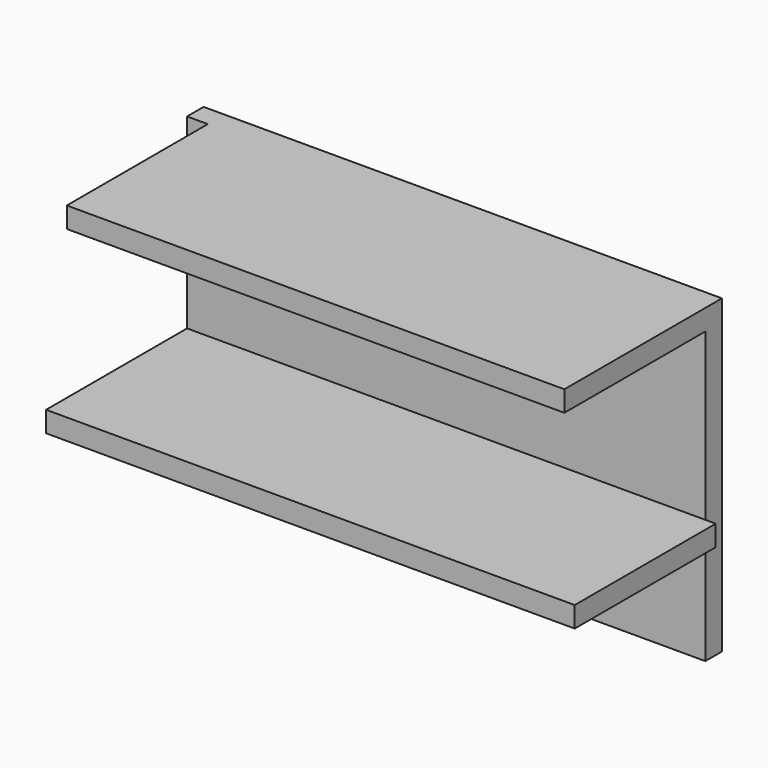
from build123d import *

# Parameters (mm, degrees)
F0_W     = 480
F0_H     = 190
F1_DEPTH = 20
F2_W     = 500
F2_H     = 300
F3_DEPTH = 20
F4_W     = 10
F4_H     = 20
F4_W_2   = 500
F5_DEPTH = 170


# Not quite as in the source:
# - the program builds the solid bodies; features that only make, move or delete a surface that nothing else refers to are left out


with BuildPart() as f1:
    # F0 (on Top) → F1 (new body)
    with BuildSketch(Plane.XY):
        with Locations((10, -95)):
            Rectangle(F0_W, F0_H)
    extrude(amount=-F1_DEPTH)

    # F2 (on Front) → F3 (join)
    with BuildSketch(Plane.XZ):
        with Locations((0, -150)):
            Rectangle(F2_W, F2_H)
    extrude(amount=F3_DEPTH)

    # F4 (on face) → F5 (join)
    with BuildSketch(Plane.XZ.offset(20)):
        with Locations((255, -190)):
            Rectangle(F4_W, F4_H)
        with Locations((0, -190)):
            Rectangle(F4_W_2, F4_H)
    extrude(amount=F5_DEPTH)


solid = f1.part
